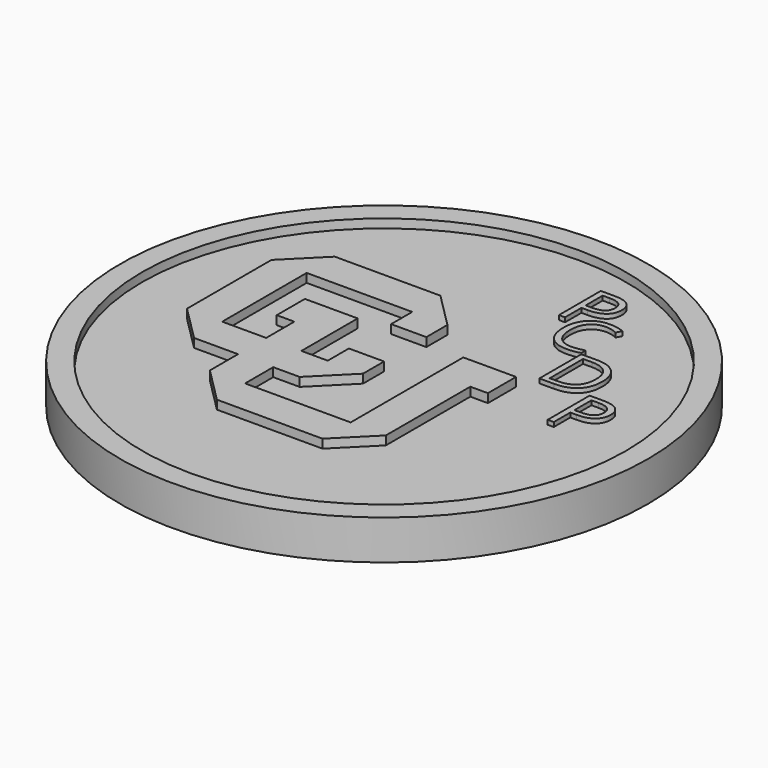
from build123d import *

# Parameters (mm, degrees)
F0_R           = 38.1
F2_DEPTH       = 3.81
F1_R           = 38.1
F1_R_2         = 34.925
F1_TEXT_SIZE   = 10.5833333333
F3_DEPTH       = 0.635
F4_R           = 38.1
F4_R_2         = 34.925
F4_TEXT_SIZE   = 12.5436938153
F4_TEXT_SIZE_2 = 11.2430837329
F4_TEXT_SIZE_3 = 11.0240065102
F5_DEPTH       = 0.635
F6_DEPTH       = 0.635
F3_FACE_R      = 38.1
F3_FACE_R_2    = 34.925
F7_DEPTH       = 0.635


# Not quite as in the source:
# - Text() gives the source's letters only with a copy of the font that has no kerning and outlines rounded to 1/6400 em; it was checked with that copy


with BuildPart() as f2:
    # F0 (on Top) → F2 (new body)
    with BuildSketch(Plane.XY):
        Circle(F0_R)
    extrude(amount=-F2_DEPTH)

    # F1 (on Top) → F3 (join)
    with BuildSketch(Plane.XY):
        Circle(F1_R)
        Circle(F1_R_2, mode=Mode.SUBTRACT)
        Polygon((0, -3.81), (0, 0), (-5.08, 0), (-5.08, -3.81), (-8.89, -3.81), (-8.89, 6.35), (-16.51, 6.35), (-16.51, 1.27), (-13.97, 1.27), (-13.97, -3.81), (-20.32, -3.81), (-20.32, 11.43), (-5.08, 11.43), (-5.08, 7.62), (0, 7.62), (0, 11.43), (-5.08, 16.51), (-20.32, 16.51), (-25.4, 11.43), (-25.4, -3.81), (-20.32, -8.89), (-13.97, -8.89), (-13.97, -13.97), (-8.89, -19.05), (6.35, -19.05), (11.43, -13.97), (11.43, 1.27), (13.97, 1.27), (13.97, 6.35), (6.35, 6.35), (6.35, -13.97), (-8.89, -13.97), (-8.89, -8.89), (-5.08, -8.89), align=None)
        with Locations((14.4526347944, 8.659887894)):
            Text('D', F1_TEXT_SIZE, font='Open Sans', text_align=(TextAlign.LEFT, TextAlign.BOTTOM))
        with Locations((6.5131504194, 22.1084709126)):
            Text('P', F1_TEXT_SIZE, font='Open Sans', text_align=(TextAlign.LEFT, TextAlign.BOTTOM))
        with Locations((21.4905514611, 1.3640065445)):
            Text('P', F1_TEXT_SIZE, font='Open Sans', text_align=(TextAlign.LEFT, TextAlign.BOTTOM))
        with Locations((9.2185150028, 16.279887894)):
            Text('C', F1_TEXT_SIZE, font='Open Sans', text_align=(TextAlign.LEFT, TextAlign.BOTTOM))
    extrude(amount=F3_DEPTH)

    # F4 (on face) + F1 (on Top) → F5 (join)
    with BuildSketch(Plane(origin=(0, 0, -3.81), x_dir=(1, 0, 0), z_dir=(0, 0, -1))):
        Circle(F4_R)
        Circle(F4_R_2, mode=Mode.SUBTRACT)
        with Locations((-25.4, 3.1706189045)):
            Text('Paulette', F4_TEXT_SIZE, font='Open Sans', font_style=FontStyle.BOLDITALIC, text_align=(TextAlign.LEFT, TextAlign.BOTTOM))
        with Locations((-19.05, -8.0950202877)):
            Text('Ozaeta', F4_TEXT_SIZE_2, font='Open Sans', font_style=FontStyle.BOLDITALIC, text_align=(TextAlign.LEFT, TextAlign.BOTTOM))
        with Locations((-12.7, -21.2414207939)):
            Text('2016', F4_TEXT_SIZE_3, font='Open Sans', font_style=FontStyle.BOLDITALIC, text_align=(TextAlign.LEFT, TextAlign.BOTTOM))
    with BuildSketch(Plane.XY):
        Circle(F1_R)
        Circle(F1_R_2, mode=Mode.SUBTRACT)
    extrude(amount=F5_DEPTH, dir=(0, 0, -1))

    # F0 (on Top) → F6 (join)
    with BuildSketch(Plane.XY):
        Circle(F0_R)
    extrude(amount=-F6_DEPTH)

    # F1 (on Top) + F3_face (on face) → F7 (join)
    with BuildSketch(Plane.XY):
        Circle(F1_R)
        Circle(F1_R_2, mode=Mode.SUBTRACT)
    with BuildSketch(Plane(origin=(-7.3089795918, -1.546462585, 0.635), x_dir=(1, 0, 0), z_dir=(0, 0, 1))):
        with Locations((7.3089795918, 1.546462585)):
            Circle(F3_FACE_R)
        with Locations((7.3089795918, 1.546462585)):
            Circle(F3_FACE_R_2, mode=Mode.SUBTRACT)
        Polygon((21.2789795918, 2.816462585), (21.2789795918, 7.896462585), (13.6589795918, 7.896462585), (13.6589795918, -12.423537415), (-1.5810204082, -12.423537415), (-1.5810204082, -7.343537415), (2.2289795918, -7.343537415), (7.3089795918, -2.263537415), (7.3089795918, 1.546462585), (2.2289795918, 1.546462585), (2.2289795918, -2.263537415), (-1.5810204082, -2.263537415), (-1.5810204082, 7.896462585), (-9.2010204082, 7.896462585), (-9.2010204082, 2.816462585), (-6.6610204082, 2.816462585), (-6.6610204082, -2.263537415), (-13.0110204082, -2.263537415), (-13.0110204082, 12.976462585), (2.2289795918, 12.976462585), (2.2289795918, 9.166462585), (7.3089795918, 9.166462585), (7.3089795918, 12.976462585), (2.2289795918, 18.056462585), (-13.0110204082, 18.056462585), (-18.0910204082, 12.976462585), (-18.0910204082, -2.263537415), (-13.0110204082, -7.343537415), (-6.6610204082, -7.343537415), (-6.6610204082, -12.423537415), (-1.5810204082, -17.503537415), (13.6589795918, -17.503537415), (18.7389795918, -12.423537415), (18.7389795918, 2.816462585), align=None)
    extrude(amount=F7_DEPTH)


solid = f2.part
